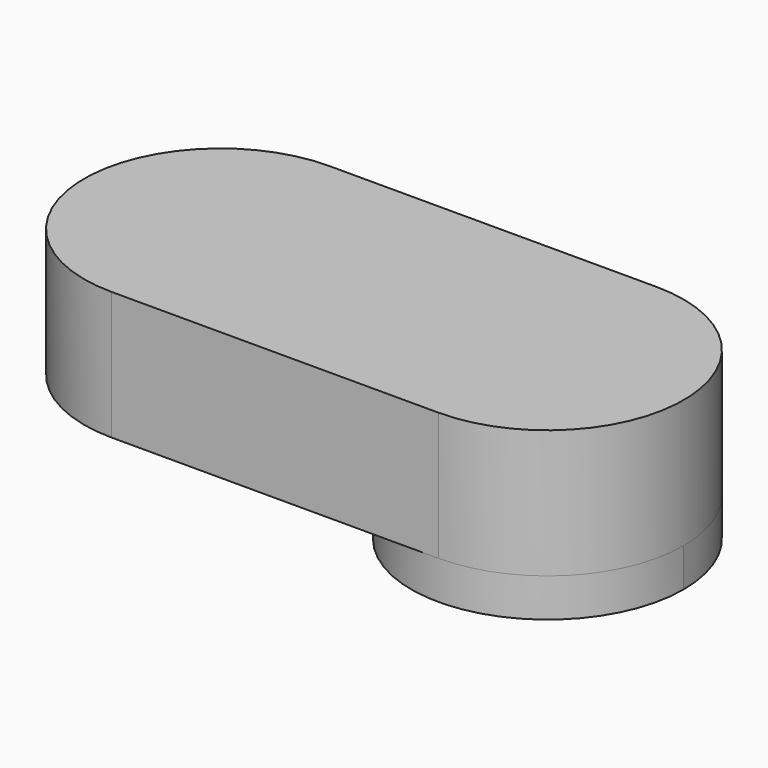
from build123d import *

# Parameters (mm, degrees)
F6_W      = 19.1
F6_H      = 8.9
F7_DEPTH  = 1.2
F10_DEPTH = 1.2
F11_R     = 2.24999
F12_W     = 19.1
F12_H     = 8.9
F13_DEPTH = 4.2
F14_DEPTH = 4
F15_W     = 19.1
F15_H     = 8.9
F16_DEPTH = 5.2


# Not quite as in the source:
# - a fillet or chamfer is up to 0.001 mm smaller than in the source, because OpenCascade refuses the exact size


with BuildPart() as f7:
    # F6 (on Top) → F7 (new body, through all)
    with BuildSketch(Plane.XY):
        with Locations((3.24578159, 0)):
            Rectangle(F6_W, F6_H)
    extrude(amount=F7_DEPTH)

    # F8 (on face) → F10 (cut, through all)
    with BuildSketch(Plane.XY.offset(1.2)):
        with BuildLine():
            Line((4.7402303145, 2.25), (-3.97921841, 2.25))
            Line((-3.97921841, 2.25), (-3.97921841, -2.25))
            Line((-3.97921841, -2.25), (4.7402303145, -2.25))
            ThreePointArc((4.7402303145, -2.25), (4.09578159, 0), (4.7402303145, 2.25))
        make_face()
        with BuildLine():
            ThreePointArc((12.59578159, 0), (9.5160181215, 4.0857124789), (4.7402303145, 2.25))
            ThreePointArc((4.7402303145, 2.25), (4.09578159, 0), (4.7402303145, -2.25))
            ThreePointArc((4.7402303145, -2.25), (9.5160181215, -4.0857124789), (12.59578159, 0))
        make_face()
    extrude(amount=-F10_DEPTH, mode=Mode.SUBTRACT)

    # F11 (radius 2.25 in the source; OpenCascade refuses exactly that, so slightly less here)
    f11_edges = [f7.edges().sort_by_distance(p)[0] for p in [
        (-3.979218, 2.25, 0.6),
        (-3.979218, -2.25, 0.6),
    ]]
    fillet(f11_edges, radius=F11_R)

    # F12 (on face) → F13 (join)
    with BuildSketch(Plane.XY.offset(1.2)):
        with Locations((3.24578159, 0)):
            Rectangle(F12_W, F12_H)
    extrude(amount=F13_DEPTH)

    # F9 (on offset) → F14 (cut, through all)
    with BuildSketch(Plane.XY.offset(1.2)):
        with BuildLine():
            Line((-1.85421841, -4.25), (8.34578159, -4.25))
            ThreePointArc((8.34578159, -4.25), (12.59578159, 0), (8.34578159, 4.25))
            Line((8.34578159, 4.25), (-1.85421841, 4.25))
            ThreePointArc((-1.85421841, 4.25), (1.15098541, 3.00520382), (2.39578159, 0))
            ThreePointArc((2.39578159, 0), (1.15098541, -3.00520382), (-1.85421841, -4.25))
        make_face()
        with BuildLine():
            ThreePointArc((-1.85421841, 4.25), (-6.10421841, 0), (-1.85421841, -4.25))
            ThreePointArc((-1.85421841, -4.25), (1.15098541, -3.00520382), (2.39578159, 0))
            ThreePointArc((2.39578159, 0), (1.15098541, 3.00520382), (-1.85421841, 4.25))
        make_face()
    extrude(amount=F14_DEPTH, mode=Mode.SUBTRACT)


with BuildPart() as f16:
    # F15 (on face) → F16 (new body, through all)
    with BuildSketch(Plane(origin=(0, 0, 0), x_dir=(1, 0, 0), z_dir=(0, 0, -1))):
        with Locations((3.24578159, 0)):
            Rectangle(F15_W, F15_H)
    extrude(amount=-F16_DEPTH)

    # F17: cut F7
    add(f7.part, mode=Mode.SUBTRACT)


solid = f16.part
